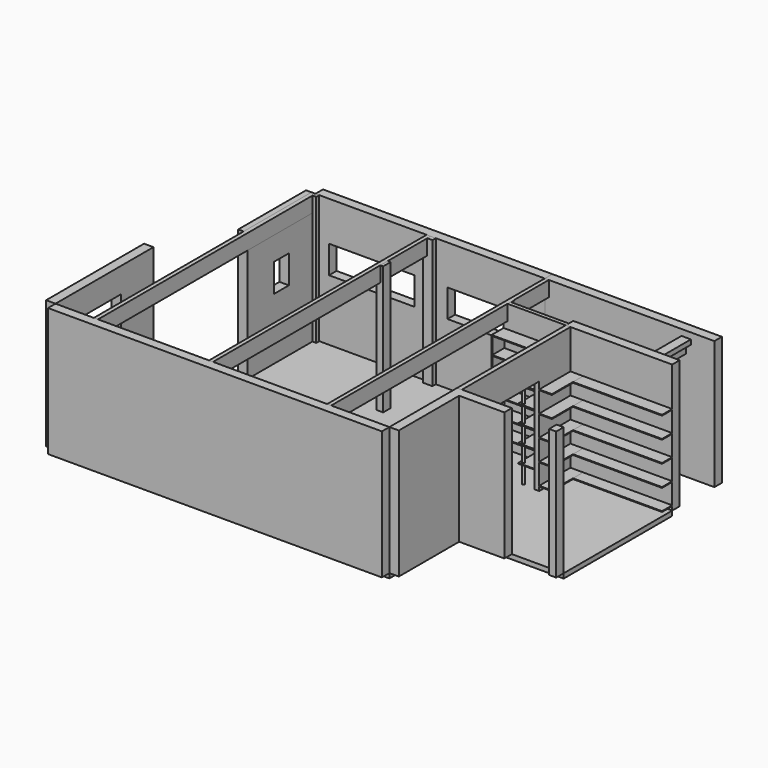
from build123d import *

# Parameters (mm, degrees)
F0_W           = 2260
F0_H           = 2880
F1_DEPTH       = 100
F3_DEPTH       = 105
F4_W           = 200
F4_H           = 2600
F5_DEPTH       = 2730
F4_H_2         = 1600
F4_H_3         = 200
F4_W_2         = 960
F4_W_3         = 7090
F4_H_4         = 1800
F4_W_4         = 6190
F4_W_5         = 150
F4_W_6         = 2260
F6_W           = 1260
F6_H           = 900
F7_DEPTH       = 210
F8_W           = 400
F8_H           = 600
F9_DEPTH       = 210
F10_W          = 80
F10_H          = 80
F11_DEPTH      = 2730
F10_W_2        = 195
F10_H_2        = 90
F10_W_3        = 145
F10_H_3        = 200
F12_W          = 1810
F12_H          = 590
F12_W_2        = 1800
F13_DEPTH      = 210
F15_DEPTH      = 100
F16_W          = 1320
F16_H          = 1287.050075531
F17_DEPTH      = 260
F18_W          = 1318.9476394653
F18_H          = 200
F19_DEPTH      = 3080
F21_DEPTH      = 2730
F23_DEPTH      = 1030
F24_W          = 3600
F24_H          = 200
F25_DEPTH      = 2730
F26_W          = 1318.3893966675
F26_H          = 16
F27_DEPTH      = 320
F28_W          = 16
F28_H          = 320
F29_DEPTH      = 2250
F31_W          = 325
F31_H          = 16
F32_DEPTH      = 535
F34_DEPTH      = 2250
F36_W          = 87
F36_H          = 325
F37_DEPTH      = 3975
F37_DEPTH_BACK = 1800
F36_W_2        = 85
F38_W          = 830
F38_H          = 16
F39_DEPTH      = 270
F40_W          = 270
F40_H          = 16
F41_DEPTH      = 1890


with BuildPart() as f1:
    # F0 (on Top) → F1 (new body)
    with BuildSketch(Plane.XY):
        Polygon((0, 5775), (0, 0), (7090, 0), (7090, 1800), (7090, 4680), (7090, 5775), align=None)
        with Locations((8220, 3240)):
            Rectangle(F0_W, F0_H)
    extrude(amount=-F1_DEPTH)

    # F2 (on face) → F3 (cut, symmetric)
    with BuildSketch(Plane.XY):
        Polygon((900, 5775), (0, 5775), (0, 2600), (900, 3975), align=None)
    extrude(amount=F3_DEPTH, both=True, mode=Mode.SUBTRACT)

    # F16 (on face) → F17 (cut)
    with BuildSketch(Plane.XY):
        with Locations((6430, 5323.5250377655)):
            Rectangle(F16_W, F16_H)
    extrude(amount=-F17_DEPTH, mode=Mode.SUBTRACT)


with BuildPart() as f5:
    # F4 (on face) → F5 (new body)
    with BuildSketch(Plane.XY):
        with Locations((-100, 1300)):
            Rectangle(F4_W, F4_H)
    extrude(amount=F5_DEPTH)

    # F6 (on face) → F7 (cut)
    with BuildSketch(Plane.YZ):
        with Locations((1110, 1750)):
            Rectangle(F6_W, F6_H)
    extrude(amount=-F7_DEPTH, mode=Mode.SUBTRACT)


with BuildPart() as f5b:
    # F4 (on face) → F5, piece 2 (new body)
    with BuildSketch(Plane.XY):
        with Locations((7190, 800)):
            Rectangle(F4_W, F4_H_2)
        with Locations((7190, 1700)):
            Rectangle(F4_W, F4_H_3)
        with Locations((7770, 1700)):
            Rectangle(F4_W_2, F4_H_3)
    extrude(amount=F5_DEPTH)


with BuildPart() as f5c:
    # F4 (on face) → F5, piece 3 (new body)
    with BuildSketch(Plane.XY):
        with Locations((3545, -100)):
            Rectangle(F4_W_3, F4_H_3)
    extrude(amount=F5_DEPTH)


with BuildPart() as f5d:
    # F4 (on face) → F5, piece 4 (new body)
    with BuildSketch(Plane.XY):
        with Locations((800, 4875)):
            Rectangle(F4_W, F4_H_4)
    extrude(amount=F5_DEPTH)

    # F8 (on face) → F9 (cut)
    with BuildSketch(Plane.YZ.offset(900)):
        with Locations((4868.8858032227, 1604.9321174622)):
            Rectangle(F8_W, F8_H)
    extrude(amount=-F9_DEPTH, mode=Mode.SUBTRACT)


with BuildPart() as f5e:
    # F4 (on face) → F5, piece 5 (new body)
    with BuildSketch(Plane.XY):
        with Locations((3995, 5875)):
            Rectangle(F4_W_4, F4_H_3)
    extrude(amount=F5_DEPTH)

    # F12 (on face) → F13 (cut)
    with BuildSketch(Plane.XZ.offset(-5775)):
        with Locations((2092.5975346565, 1595)):
            Rectangle(F12_W, F12_H)
        with Locations((4603.2698345184, 1595)):
            Rectangle(F12_W_2, F12_H)
    extrude(amount=-F13_DEPTH, mode=Mode.SUBTRACT)

    # F18 (on face) → F19 (cut)
    with BuildSketch(Plane(origin=(0, 0, 0), x_dir=(1, 0, 0), z_dir=(0, 0, -1))):
        with Locations((6430.5261802673, -5875)):
            Rectangle(F18_W, F18_H)
    extrude(amount=-F19_DEPTH, mode=Mode.SUBTRACT)


with BuildPart() as f5f:
    # F4 (on face) → F5, piece 6 (new body)
    with BuildSketch(Plane.XY):
        with Locations((9275, 1700)):
            Rectangle(F4_W_5, F4_H_3)
    extrude(amount=F5_DEPTH)


with BuildPart() as f5g:
    # F4 (on face) → F5, piece 7 (new body)
    with BuildSketch(Plane.XY):
        with Locations((8220, 4780)):
            Rectangle(F4_W_6, F4_H_3)
    extrude(amount=F5_DEPTH)

    # F22 (on face) → F23 (join)
    with BuildSketch(Plane.XZ.offset(-5775)):
        Polygon((6271.0523605347, 0), (5771.0523605347, 0), (5771.0523605347, -100.0000238419), (6371.0523843765, -100.0000238419), (6371.0523843765, 99.9999761581), (6571.0523843765, 99.9999761581), (6571.0523843765, 299.9999761581), (6771.0523843765, 299.9999761581), (6771.0523843765, 499.9999761581), (6971.0523843765, 499.9999761581), (6971.0523843765, 699.9999761581), (7171.0523843765, 699.9999761581), (7171.0523843765, 899.9999761581), (7371.0523843765, 899.9999761581), (7371.0523843765, 1099.9999761581), (7571.0523843765, 1099.9999761581), (7571.0523843765, 1299.9999761581), (7771.0523843765, 1299.9999761581), (7771.0523843765, 1499.9999761581), (7971.0523843765, 1499.9999761581), (7971.0523843765, 1699.9999761581), (8171.0523843765, 1699.9999761581), (8171.0523843765, 1899.9999761581), (8371.0523843765, 1899.9999761581), (8371.0523843765, 2099.9999761581), (8571.0523843765, 2099.9999761581), (8571.0523843765, 2299.9999761581), (8771.0523843765, 2299.9999761581), (8771.0523843765, 2499.9999761581), (8871.0523605347, 2499.9999761581), (8871.0523605347, 2600), (8671.0523605347, 2600), (8671.0523605347, 2400), (8471.0523605347, 2400), (8471.0523605347, 2200), (8271.0523605347, 2200), (8271.0523605347, 2000), (8071.0523605347, 2000), (8071.0523605347, 1800), (7871.0523605347, 1800), (7871.0523605347, 1600), (7671.0523605347, 1600), (7671.0523605347, 1400), (7471.0523605347, 1400), (7471.0523605347, 1200), (7271.0523605347, 1200), (7271.0523605347, 1000), (7071.0523605347, 1000), (7071.0523605347, 800), (6871.0523605347, 800), (6871.0523605347, 600), (6671.0523605347, 600), (6671.0523605347, 400), (6471.0523605347, 400), (6471.0523605347, 200), (6271.0523605347, 200), align=None)
    extrude(amount=F23_DEPTH)


with BuildPart() as f11:
    # F10 (on face) → F11 (new body)
    with BuildSketch(Plane.XY):
        with Locations((940, 5735)):
            Rectangle(F10_W, F10_H)
    extrude(amount=F11_DEPTH)


with BuildPart() as f11b:
    # F10 (on face) → F11, piece 2 (new body)
    with BuildSketch(Plane.XY):
        with Locations((3357.5, 5730)):
            Rectangle(F10_W_2, F10_H_2)
    extrude(amount=F11_DEPTH)


with BuildPart() as f11c:
    # F10 (on face) → F11, piece 3 (new body)
    with BuildSketch(Plane.XY):
        with Locations((3332.5, 4540)):
            Rectangle(F10_W_3, F10_H_3)
    extrude(amount=F11_DEPTH)


with BuildPart() as f15:
    # F14 (on face) → F15 (new body)
    with BuildSketch(Plane(origin=(7090, 0, 0), x_dir=(0, -1, 0), z_dir=(-1, 0, 0))):
        Polygon((-4680, 2730), (-4680, 0), (-3850, 0), (-3850, 2050), (-1794.2402362823, 2050), (-1794.2402362823, 2730), align=None)
    extrude(amount=-F15_DEPTH)


with BuildPart() as f21:
    # F20 (on face) → F21 (new body)
    with BuildSketch(Plane.XY):
        Polygon((5870, 4845), (5770, 4845), (5770, 4680), (7088.3893966675, 4680), (7088.3893966675, 4761.1832618713), (5870, 4761.1832618713), align=None)
    extrude(amount=F21_DEPTH)

    # F26 (on face) → F27 (join)
    with BuildSketch(Plane.XZ.offset(-4680)):
        with Locations((6429.1946983337, 2242)):
            Rectangle(F26_W, F26_H)
        with Locations((6429.1946983337, 1872)):
            Rectangle(F26_W, F26_H)
        with Locations((6429.1946983337, 1502)):
            Rectangle(F26_W, F26_H)
        with Locations((6429.1946983337, 1132)):
            Rectangle(F26_W, F26_H)
        with Locations((6429.1946983337, 762)):
            Rectangle(F26_W, F26_H)
        with Locations((6429.1946983337, 392)):
            Rectangle(F26_W, F26_H)
    extrude(amount=F27_DEPTH)


with BuildPart() as f25:
    # F24 (on face) → F25 (new body)
    with BuildSketch(Plane.XY):
        with Locations((7570, 5875)):
            Rectangle(F24_W, F24_H)
    extrude(amount=F25_DEPTH)


with BuildPart() as f29:
    # F28 (on face) → F29 (new body)
    with BuildSketch(Plane.XY):
        with Locations((5778, 4520)):
            Rectangle(F28_W, F28_H)
    extrude(amount=F29_DEPTH)


with BuildPart() as f32:
    # F31 (on offset) → F32 (new body, through all)
    with BuildSketch(Plane.XZ.offset(-3825)):
        with Locations((6927.5, 2242)):
            Rectangle(F31_W, F31_H)
    extrude(amount=-F32_DEPTH)


with BuildPart() as f32b:
    # F31 (on offset) → F32, piece 2 (new body, through all)
    with BuildSketch(Plane.XZ.offset(-3825)):
        with Locations((6927.5, 1872)):
            Rectangle(F31_W, F31_H)
    extrude(amount=-F32_DEPTH)


with BuildPart() as f32c:
    # F31 (on offset) → F32, piece 3 (new body, through all)
    with BuildSketch(Plane.XZ.offset(-3825)):
        with Locations((6927.5, 1502)):
            Rectangle(F31_W, F31_H)
    extrude(amount=-F32_DEPTH)


with BuildPart() as f32d:
    # F31 (on offset) → F32, piece 4 (new body, through all)
    with BuildSketch(Plane.XZ.offset(-3825)):
        with Locations((6927.5, 1132)):
            Rectangle(F31_W, F31_H)
    extrude(amount=-F32_DEPTH)


with BuildPart() as f32e:
    # F31 (on offset) → F32, piece 5 (new body, through all)
    with BuildSketch(Plane.XZ.offset(-3825)):
        with Locations((6927.5, 762)):
            Rectangle(F31_W, F31_H)
    extrude(amount=-F32_DEPTH)


with BuildPart() as f32f:
    # F31 (on offset) → F32, piece 6 (new body, through all)
    with BuildSketch(Plane.XZ.offset(-3825)):
        with Locations((6927.5, 392)):
            Rectangle(F31_W, F31_H)
    extrude(amount=-F32_DEPTH)


with BuildPart() as f34:
    # F33 (on face) → F34 (new body)
    with BuildSketch(Plane.XY.offset(2250)):
        Polygon((6824.29066821, 3916.0963969695), (6793.8232421875, 3882.9793930054), (6826.9402461516, 3852.5119669828), (6857.4076721742, 3885.628970947), align=None)
    extrude(amount=-F34_DEPTH)


with BuildPart() as f37:
    # F36 (on face) → F37 (new body, two sides)
    with BuildSketch(Plane.XZ.offset(-3975)) as f37_sk:
        with Locations((858.5, 2567.5)):
            Rectangle(F36_W, F36_H)
    extrude(amount=F37_DEPTH)
    extrude(f37_sk.sketch, amount=-F37_DEPTH_BACK)


with BuildPart() as f37b:
    # F36 (on face) → F37, piece 2 (new body, two sides)
    with BuildSketch(Plane.XZ.offset(-3975)) as f37_2_sk:
        with Locations((3302.5581645966, 2567.5)):
            Rectangle(F36_W_2, F36_H)
    extrude(amount=F37_DEPTH)
    extrude(f37_2_sk.sketch, amount=-F37_DEPTH_BACK)


with BuildPart() as f37c:
    # F36 (on face) → F37, piece 3 (new body, two sides)
    with BuildSketch(Plane.XZ.offset(-3975)) as f37_3_sk:
        with Locations((5811.3140869141, 2567.5)):
            Rectangle(F36_W_2, F36_H)
    extrude(amount=F37_DEPTH)
    extrude(f37_3_sk.sketch, amount=-F37_DEPTH_BACK)


with BuildPart() as f39:
    # F38 (on face) → F39 (new body)
    with BuildSketch(Plane.YZ.offset(7190)):
        with Locations((4265, 1892)):
            Rectangle(F38_W, F38_H)
    extrude(amount=F39_DEPTH)


with BuildPart() as f39b:
    # F38 (on face) → F39, piece 2 (new body)
    with BuildSketch(Plane.YZ.offset(7190)):
        with Locations((4265, 1442)):
            Rectangle(F38_W, F38_H)
    extrude(amount=F39_DEPTH)


with BuildPart() as f39c:
    # F38 (on face) → F39, piece 3 (new body)
    with BuildSketch(Plane.YZ.offset(7190)):
        with Locations((4265, 992)):
            Rectangle(F38_W, F38_H)
    extrude(amount=F39_DEPTH)


with BuildPart() as f39d:
    # F38 (on face) → F39, piece 4 (new body)
    with BuildSketch(Plane.YZ.offset(7190)):
        with Locations((4265, 542)):
            Rectangle(F38_W, F38_H)
    extrude(amount=F39_DEPTH)


with BuildPart() as f39e:
    # F38 (on face) → F39, piece 5 (new body)
    with BuildSketch(Plane.YZ.offset(7190)):
        with Locations((4265, 92)):
            Rectangle(F38_W, F38_H)
    extrude(amount=F39_DEPTH)


with BuildPart() as f41:
    # F40 (on face) → F41 (new body, through all)
    with BuildSketch(Plane.YZ.offset(9350)):
        with Locations((4545, 1892)):
            Rectangle(F40_W, F40_H)
    extrude(amount=-F41_DEPTH)


with BuildPart() as f41b:
    # F40 (on face) → F41, piece 2 (new body, through all)
    with BuildSketch(Plane.YZ.offset(9350)):
        with Locations((4545, 1442)):
            Rectangle(F40_W, F40_H)
    extrude(amount=-F41_DEPTH)


with BuildPart() as f41c:
    # F40 (on face) → F41, piece 3 (new body, through all)
    with BuildSketch(Plane.YZ.offset(9350)):
        with Locations((4545, 992)):
            Rectangle(F40_W, F40_H)
    extrude(amount=-F41_DEPTH)


with BuildPart() as f41d:
    # F40 (on face) → F41, piece 4 (new body, through all)
    with BuildSketch(Plane.YZ.offset(9350)):
        with Locations((4545, 542)):
            Rectangle(F40_W, F40_H)
    extrude(amount=-F41_DEPTH)


with BuildPart() as f41e:
    # F40 (on face) → F41, piece 5 (new body, through all)
    with BuildSketch(Plane.YZ.offset(9350)):
        with Locations((4545, 92)):
            Rectangle(F40_W, F40_H)
    extrude(amount=-F41_DEPTH)


solid = Compound([f1.part, f5.part, f5b.part, f5c.part, f5d.part, f5e.part, f5f.part, f5g.part, f11.part, f11b.part, f11c.part, f15.part, f21.part, f25.part, f29.part, f32.part, f32b.part, f32c.part, f32d.part, f32e.part, f32f.part, f34.part, f37.part, f37b.part, f37c.part, f39.part, f39b.part, f39c.part, f39d.part, f39e.part, f41.part, f41b.part, f41c.part, f41d.part, f41e.part])
